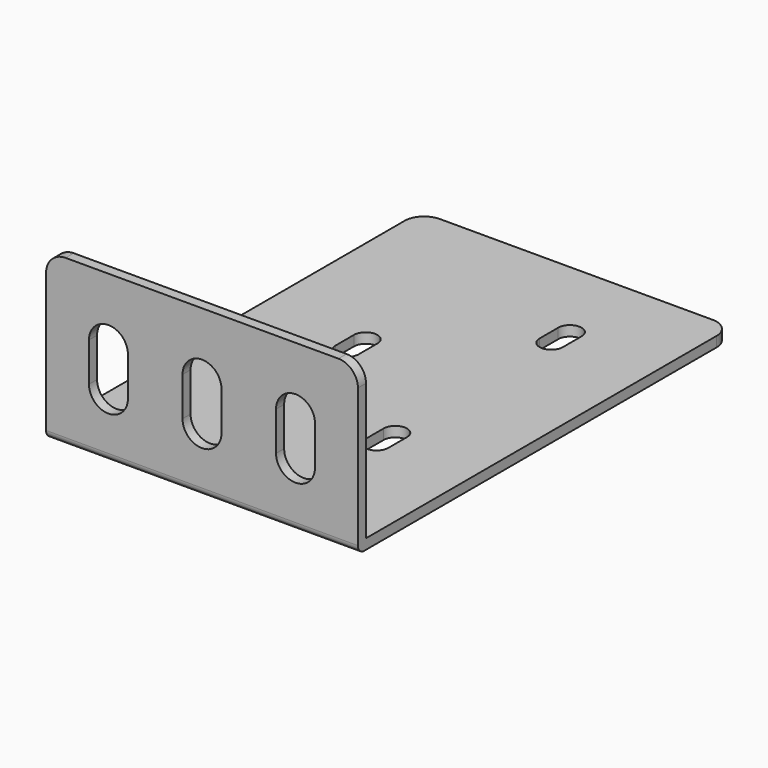
from build123d import *

# Parameters (mm, degrees)
F0_W     = 50.8
F0_H     = 76.2
F1_DEPTH = 1.651
F2_W     = 50.8
F2_H     = 1.651
F3_DEPTH = 25.4
F4_R     = 1.27
F5_R     = 3.175
F6_W     = 1.905
F6_H     = 3.81
F7_DEPTH = 25.4
F9_DEPTH = 25.4


# Not quite as in the source:
# - a feature names something its author has since deleted; it is built from what else it names


with BuildPart() as f1:
    # F0 (on Top) → F1 (new body)
    with BuildSketch(Plane.XY):
        with Locations((0, -3.81)):
            Rectangle(F0_W, F0_H)
    extrude(amount=F1_DEPTH)

    # F2 (on face) → F3 (join)
    with BuildSketch(Plane.XY.offset(1.651)):
        with Locations((0, -41.0845)):
            Rectangle(F2_W, F2_H)
    extrude(amount=F3_DEPTH)

    # F4
    f4_edges = [f1.edges().sort_by_distance(p)[0] for p in [
        (0, -41.91, 0),
    ]]
    fillet(f4_edges, radius=F4_R)

    # F5
    f5_edges = [f1.edges().sort_by_distance(p)[0] for p in [
        (25.4, 34.29, 0.8255),
        (-25.4, 34.29, 0.8255),
        (25.4, -41.0845, 27.051),
        (-25.4, -41.0845, 27.051),
    ]]
    fillet(f5_edges, radius=F5_R)

    # F6 (on face) → F7 (cut)
    with BuildSketch(Plane.XY.offset(1.651)):
        with BuildLine():
            Line((-6.985, -1.27), (-6.985, 2.54))
            ThreePointArc((-6.985, 2.54), (-8.89, 4.445), (-10.795, 2.54))
            Line((-10.795, 2.54), (-8.89, 2.54))
            Line((-8.89, 2.54), (-8.89, -1.27))
            Line((-8.89, -1.27), (-10.795, -1.27))
            ThreePointArc((-10.795, -1.27), (-8.89, -3.175), (-6.985, -1.27))
        make_face()
        with Locations((-9.8425, 0.635)):
            Rectangle(F6_W, F6_H)
        with BuildLine():
            ThreePointArc((8.255, 16.51), (10.16, 14.605), (12.065, 16.51))
            Line((12.065, 16.51), (12.065, 20.32))
            ThreePointArc((12.065, 20.32), (10.16, 22.225), (8.255, 20.32))
            Line((8.255, 20.32), (8.255, 16.51))
        make_face()
        with BuildLine():
            ThreePointArc((12.065, -15.24), (10.16, -13.335), (8.255, -15.24))
            Line((8.255, -15.24), (8.255, -19.05))
            ThreePointArc((8.255, -19.05), (10.16, -20.955), (12.065, -19.05))
            Line((12.065, -19.05), (12.065, -15.24))
        make_face()
    extrude(amount=-F7_DEPTH, mode=Mode.SUBTRACT)

    # F8 (on face) → F9 (cut)
    with BuildSketch(Plane.XZ.offset(41.91)):
        with BuildLine():
            ThreePointArc((-12.065, 16.51), (-15.24, 19.685), (-18.415, 16.51))
            Line((-18.415, 16.51), (-18.415, 10.16))
            ThreePointArc((-18.415, 10.16), (-15.24, 6.985), (-12.065, 10.16))
            Line((-12.065, 10.16), (-12.065, 16.51))
        make_face()
        with BuildLine():
            Line((3.175, 10.16), (3.175, 16.51))
            ThreePointArc((3.175, 16.51), (0, 19.685), (-3.175, 16.51))
            Line((-3.175, 16.51), (-3.175, 10.16))
            ThreePointArc((-3.175, 10.16), (0, 6.985), (3.175, 10.16))
        make_face()
        with BuildLine():
            Line((18.415, 10.16), (18.415, 16.51))
            ThreePointArc((18.415, 16.51), (15.24, 19.685), (12.065, 16.51))
            Line((12.065, 16.51), (12.065, 10.16))
            ThreePointArc((12.065, 10.16), (15.24, 6.985), (18.415, 10.16))
        make_face()
    extrude(amount=-F9_DEPTH, mode=Mode.SUBTRACT)


solid = f1.part
